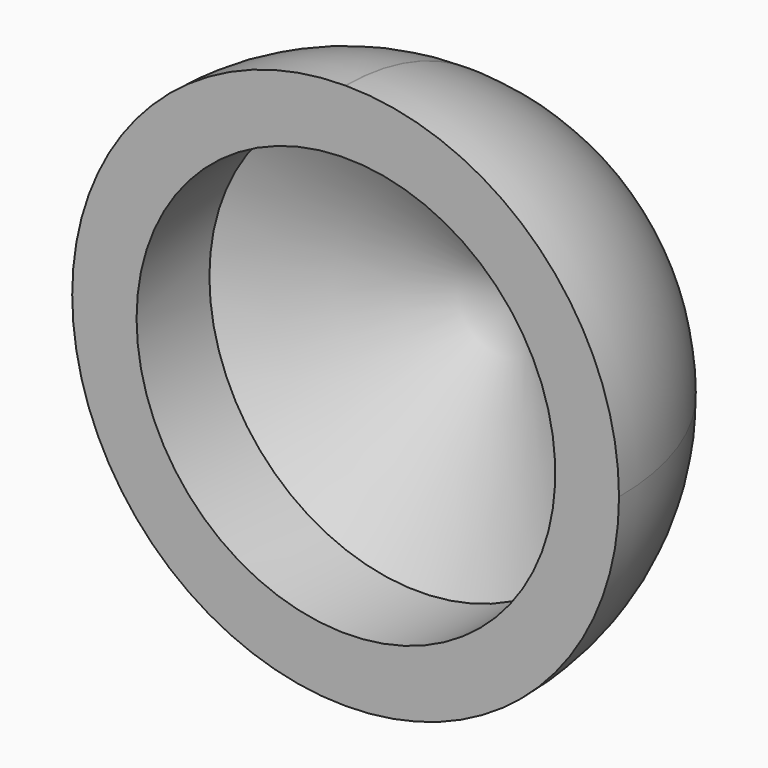
from build123d import *

# Parameters (mm, degrees)
F0_W     = 76.2886069715
F0_H     = 38.1443030201
F1_DEPTH = 76.2
F2_R     = 38.09999
F4_R     = 38.09999
F5_D     = 58.42
F5_DEPTH = 12.7
F5_TIP   = 17.5511386818


# Not quite as in the source:
# - a fillet or chamfer is up to 0.001 mm smaller than in the source, because OpenCascade refuses the exact size


with BuildPart() as f1:
    # F0 (on Top) → F1 (new body)
    with BuildSketch(Plane.XY):
        with Locations((-1.9769910723, 14.3041138072)):
            Rectangle(F0_W, F0_H)
    extrude(amount=F1_DEPTH)

    # F2 (radius 38.1 in the source; OpenCascade refuses exactly that, so slightly less here)
    f2_edges = [f1.edges().sort_by_distance(p)[0] for p in [
        (-40.121295, 14.304114, 76.2),
        (-40.121295, 14.304114, 0),
        (36.167312, 14.304114, 0),
        (36.167312, 14.304114, 76.2),
    ]]
    fillet(f2_edges, radius=F2_R)

    # F4 (radius 38.1 in the source; OpenCascade refuses exactly that, so slightly less here)
    f4_edges = [f1.edges().sort_by_distance(p)[0] for p in [
        (-28.962066, 33.376265, 11.159229),
        (25.008084, 33.376265, 11.159229),
    ]]
    fillet(f4_edges, radius=F4_R)

    # F5
    with Locations(Plane.XZ.offset(4.7680377029)):
        with Locations((-1.9326875865, 38.1)):
            Hole(F5_D / 2, depth=F5_DEPTH)
            with Locations((0, 0, -(F5_DEPTH + F5_TIP / 2))):  # 118° drill point
                Cone(0, F5_D / 2, F5_TIP, mode=Mode.SUBTRACT)


solid = f1.part
